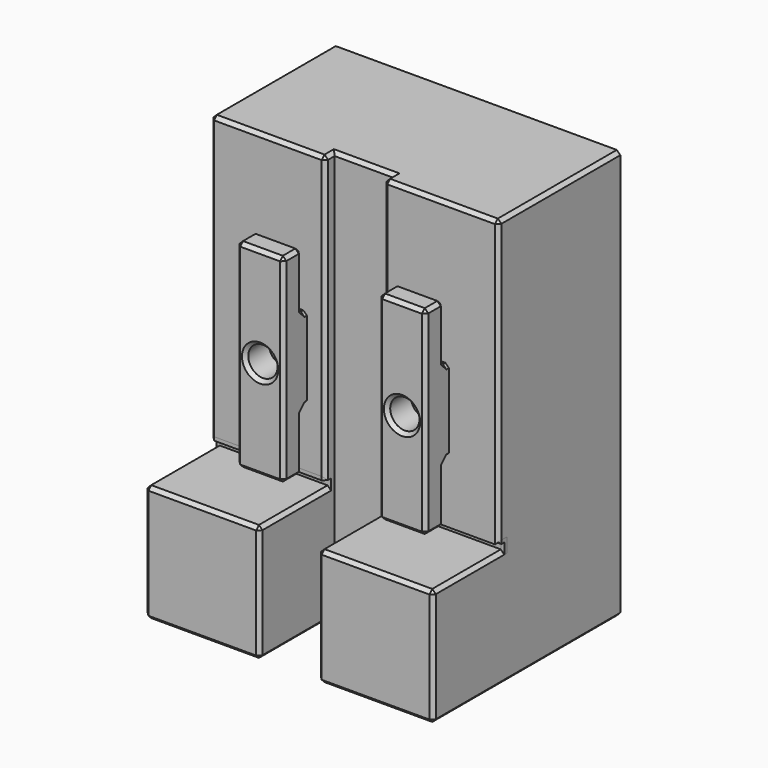
from build123d import *

# Parameters (mm, degrees)
F1_DEPTH  = 44.45
F2_W      = 12.446
F2_H      = 8.89
F3_DEPTH  = 31.75
F4_W      = 0.7874
F4_H      = 0.7874
F5_DEPTH  = 31.243
F6_SIZE   = 0.381
F8_D      = 2.2606
F8_DEPTH  = 12.7
F8_TIP    = 0.6791527577
F9_W      = 5.08
F9_H      = 21.5646
F9_R      = 1.5875
F10_DEPTH = 3.175
F11_W     = 0.7112
F11_H     = 6.35
F12_DEPTH = 25.8582
F13_SIZE  = 0.381
F14_W     = 42.4513401179
F14_H     = 23.650664404
F15_DEPTH = 44.451


with BuildPart() as f1:
    # F0 (on Top) → F1 (new body)
    with BuildSketch(Plane.XY):
        Polygon((15.621, -19.05), (15.621, 19.05), (3.175, 19.05), (3.175, 8.89), (-3.175, 8.89), (-3.175, 19.05), (-15.621, 19.05), (-15.621, -19.05), (-3.175, -19.05), (-3.175, -8.89), (3.175, -8.89), (3.175, -19.05), align=None)
    extrude(amount=F1_DEPTH)

    # F2 (on face) → F3 (cut)
    with BuildSketch(Plane.XY.offset(44.45)):
        with Locations((-9.398, -14.605)):
            Rectangle(F2_W, F2_H)
        with Locations((9.398, -14.605)):
            Rectangle(F2_W, F2_H)
        with Locations((9.398, 14.605)):
            Rectangle(F2_W, F2_H)
        with Locations((-9.398, 14.605)):
            Rectangle(F2_W, F2_H)
    extrude(amount=-F3_DEPTH, mode=Mode.SUBTRACT)

    # F4 (on face) → F5 (cut, through all)
    with BuildSketch(Plane.YZ.offset(15.621)):
        with Locations((-9.7663, 13.0937)):
            Rectangle(F4_W, F4_H)
        with Locations((9.7663, 13.0937)):
            Rectangle(F4_W, F4_H)
    extrude(amount=-F5_DEPTH, mode=Mode.SUBTRACT)

    # F6
    f6_edges = [f1.edges().sort_by_distance(p)[0] for p in [
        (9.398, 10.16, 44.45),
        (15.621, 10.16, 28.9687),
        (9.398, 10.16, 13.4874),
        (3.175, 10.16, 28.9687),
        (-9.398, 10.16, 44.45),
        (-3.175, 10.16, 28.9687),
        (-9.398, 10.16, 13.4874),
        (-15.621, 10.16, 28.9687),
        (-9.398, 19.05, 0),
        (-15.621, 19.05, 6.35),
        (-9.398, 19.05, 12.7),
        (-3.175, 19.05, 6.35),
        (9.398, 19.05, 0),
        (3.175, 19.05, 6.35),
        (9.398, 19.05, 12.7),
        (15.621, 19.05, 6.35),
        (-15.621, 0, 0),
        (-15.621, 14.2113, 12.7),
        (-15.621, 9.3726, 13.0937),
        (-15.621, 9.7663, 13.4874),
        (-15.621, 0, 44.45),
        (-15.621, -10.16, 28.9687),
        (-15.621, -9.7663, 13.4874),
        (-15.621, -9.3726, 13.0937),
        (-15.621, -14.2113, 12.7),
        (-15.621, -19.05, 6.35),
        (9.398, -10.16, 44.45),
        (3.175, -10.16, 28.9687),
        (9.398, -10.16, 13.4874),
        (15.621, -10.16, 28.9687),
        (9.398, -19.05, 0),
        (15.621, -19.05, 6.35),
        (9.398, -19.05, 12.7),
        (3.175, -19.05, 6.35),
        (-9.398, -19.05, 0),
        (-3.175, -19.05, 6.35),
        (-9.398, -19.05, 12.7),
        (15.621, 0, 0),
        (3.175, 13.97, 0),
        (0, 8.89, 0),
        (-3.175, 13.97, 0),
        (-3.175, -13.97, 0),
        (0, -8.89, 0),
        (3.175, -13.97, 0),
        (3.175, -9.525, 44.45),
        (0, -8.89, 44.45),
        (-3.175, -9.525, 44.45),
        (-9.398, -10.16, 44.45),
        (-3.175, 9.525, 44.45),
        (0, 8.89, 44.45),
        (3.175, 9.525, 44.45),
        (15.621, 0, 44.45),
        (-3.175, -14.2113, 12.7),
        (3.175, -14.2113, 12.7),
        (3.175, 14.2113, 12.7),
        (-3.175, 14.2113, 12.7),
        (15.621, -14.2113, 12.7),
        (-3.175, -10.16, 28.9687),
        (15.621, 14.2113, 12.7),
    ]]
    chamfer(f6_edges, length=F6_SIZE)

    # F8
    with Locations(Plane.XZ.offset(10.16)):
        with Locations((7.6962, 24.638)):
            Hole(F8_D / 2, depth=F8_DEPTH)
            with Locations((0, 0, -(F8_DEPTH + F8_TIP / 2))):  # 118° drill point
                Cone(0, F8_D / 2, F8_TIP, mode=Mode.SUBTRACT)

    # F14 (on face) → F15 (cut, through all)
    with BuildSketch(Plane(origin=(0, 0, 0), x_dir=(1, 0, 0), z_dir=(0, 0, -1))):
        with Locations((-0.5870210007, -18.175332202)):
            Rectangle(F14_W, F14_H)
    extrude(amount=-F15_DEPTH, mode=Mode.SUBTRACT)


with BuildPart() as f10:
    # F9 (on face) → F10 (new body)
    with BuildSketch(Plane.XZ.offset(10.16)):
        with Locations((7.6962, 24.6507)):
            Rectangle(F9_W, F9_H)
        with Locations((7.6962, 24.638)):
            Circle(F9_R, mode=Mode.SUBTRACT)
    extrude(amount=F10_DEPTH)

    # F11 (on face) → F12 (cut, through all)
    with BuildSketch(Plane.YZ.offset(10.2362)):
        with Locations((-10.5156, 17.0434)):
            Rectangle(F11_W, F11_H)
        with Locations((-10.5156, 32.258)):
            Rectangle(F11_W, F11_H)
    extrude(amount=-F12_DEPTH, mode=Mode.SUBTRACT)

    # F13
    f13_edges = [f10.edges().sort_by_distance(p)[0] for p in [
        (10.2362, -13.335, 24.6507),
        (7.6962, -13.335, 35.433),
        (5.1562, -13.335, 24.6507),
        (7.6962, -13.335, 13.8684),
        (6.1087, -13.335, 24.638),
        (7.6962, -10.8712, 35.433),
        (5.1562, -12.1031, 35.433),
        (10.2362, -12.1031, 35.433),
        (10.2362, -10.8712, 17.0434),
        (7.6962, -10.8712, 13.8684),
        (5.1562, -10.8712, 17.0434),
        (7.6962, -10.8712, 20.2184),
        (10.2362, -10.8712, 32.258),
        (7.6962, -10.8712, 29.083),
        (5.1562, -10.8712, 32.258),
        (10.2362, -10.5156, 20.2184),
        (10.2362, -10.5156, 29.083),
        (10.2362, -12.1031, 13.8684),
        (5.1562, -10.5156, 20.2184),
        (5.1562, -10.5156, 29.083),
        (5.1562, -12.1031, 13.8684),
    ]]
    chamfer(f13_edges, length=F13_SIZE)


with BuildPart() as f16_1:
    # F16: instance of F10
    add(f10.part.mirror(Plane.YZ))


with BuildPart() as f16_2:
    # F16: instance of F1
    add(f1.part.mirror(Plane.YZ))


solid = Compound([f1.part, f10.part, f16_1.part, f16_2.part])
